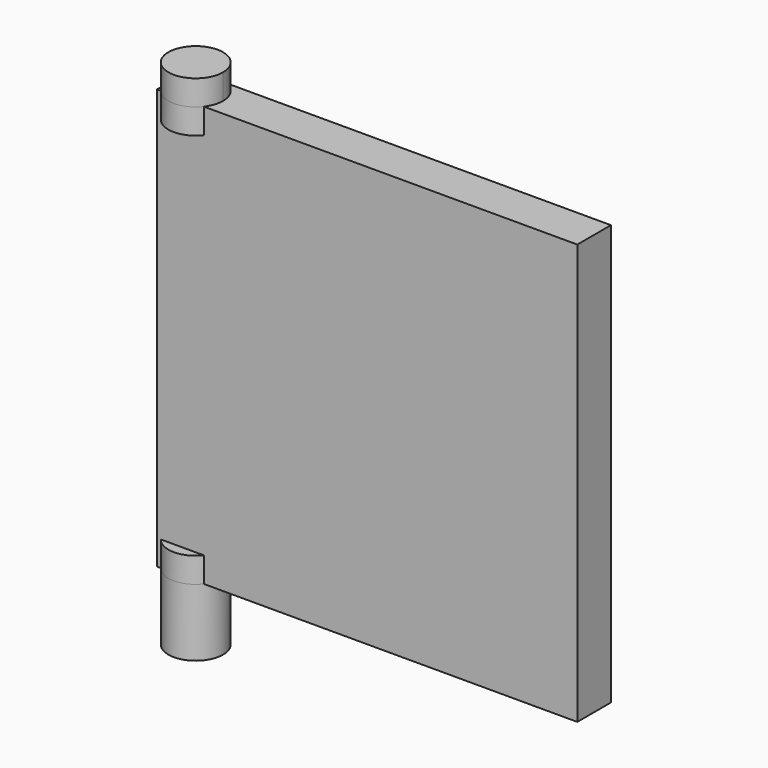
from build123d import *

# Parameters (mm, degrees)
F0_W          = 50
F0_H          = 50
F1_DEPTH      = 5
F2_R          = 3.25
F3_DEPTH      = 8
F3_DEPTH_BACK = 3
F4_R          = 3.25
F5_DEPTH      = 3
F5_DEPTH_BACK = 3
F6_T4_DEPTH   = 60
F6_S5_R       = 3.25
F6_T6_DEPTH   = 32
F6_T10_DEPTH  = 60


# Not quite as in the source:
# - a fillet or chamfer that OpenCascade refuses, or shapes differently, is made with other operations: its cross-section is extruded or revolved along the edge and cut away or added


with BuildPart() as f1:
    # F0 (on Front) → F1 (new body)
    with BuildSketch(Plane.XZ):
        with Locations((25, 25)):
            Rectangle(F0_W, F0_H)
    extrude(amount=F1_DEPTH)

    # F2 (on face) → F3 (join, two sides)
    with BuildSketch(Plane(origin=(0, 0, 0), x_dir=(1, 0, 0), z_dir=(0, 0, -1))) as f3_sk:
        with Locations((3, 3)):
            Circle(F2_R)
    extrude(amount=F3_DEPTH)
    extrude(f3_sk.sketch, amount=-F3_DEPTH_BACK)

    # F4 (on face) → F5 (join, two sides)
    with BuildSketch(Plane.XY.offset(50)) as f5_sk:
        with Locations((3, -3)):
            Circle(F4_R)
    extrude(amount=F5_DEPTH)
    extrude(f5_sk.sketch, amount=-F5_DEPTH_BACK)

    # F6: fillet of radius 2 on 1 edges, made by hand


with BuildPart() as f6_tool2:
    # F6_s3 → F6_t4 (new body)
    with BuildSketch(Plane.XY.offset(55)):
        with BuildLine():
            ThreePointArc((0, -2), (0.5857864376, -0.5857864376), (2, 0))
            Line((2, 0), (0, 0))
            Line((0, 0), (0, -2))
        make_face()
    extrude(amount=-F6_T4_DEPTH)

    # F6_s5 → F6_t6 (cut, symmetric)
    with BuildSketch(Plane.XY.offset(25)):
        with Locations((3, -3)):
            Circle(F6_S5_R)
    extrude(amount=F6_T6_DEPTH, both=True, mode=Mode.SUBTRACT)


with BuildPart() as f1_1:
    add(f1.part)

    # F6_t1: cut F6_tool2
    add(f6_tool2.part, mode=Mode.SUBTRACT)


with BuildPart() as f6_tool8:
    # F6_s9 → F6_t10 (new body)
    with BuildSketch(Plane.XY.offset(55)):
        with BuildLine():
            ThreePointArc((0, -2), (0.5857864376, -0.5857864376), (2, 0))
            Line((2, 0), (0, 0))
            Line((0, 0), (0, -2))
        make_face()
    extrude(amount=-F6_T10_DEPTH)

    split(bisect_by=Plane.XY.offset(3), keep=Keep.TOP)

    split(bisect_by=Plane.XY.offset(47), keep=Keep.BOTTOM)


with BuildPart() as f1_2:
    add(f1_1.part)

    # F6_t7: cut F6_tool8
    add(f6_tool8.part, mode=Mode.SUBTRACT)


solid = f1_2.part
